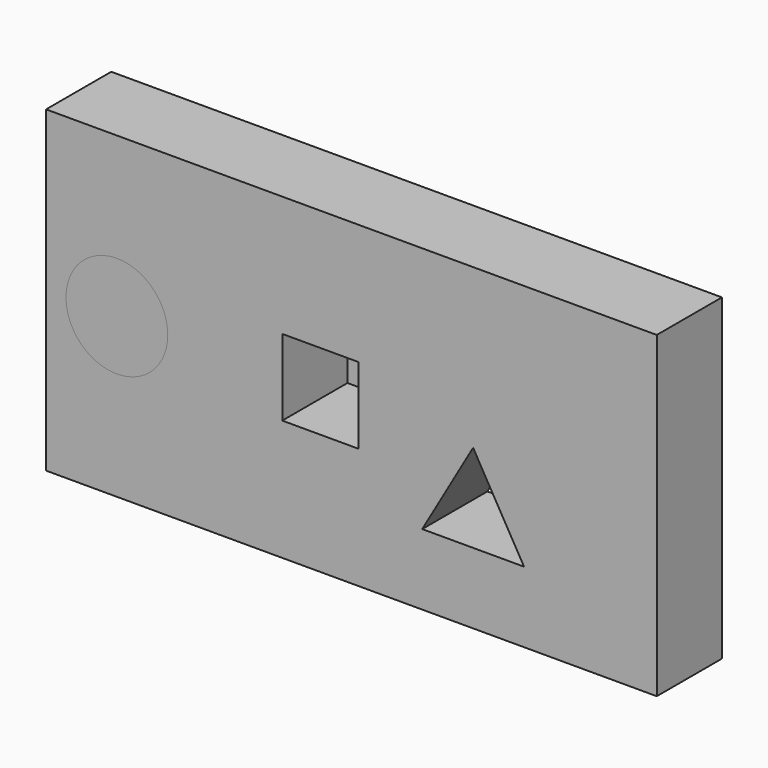
from build123d import *

# Parameters (mm, degrees)
F0_W     = 152.4
F0_H     = 79.375
F0_R     = 12.7
F0_W_2   = 19.05
F0_H_2   = 19.05
F1_DEPTH = 20.32
F2_DEPTH = 31.75
F3_DEPTH = 31.75
F4_DEPTH = 20.32


with BuildPart() as f1:
    # F0 (on Front) → F1 (new body)
    with BuildSketch(Plane.XZ):
        with Locations((-24.0162322402, 0)):
            Rectangle(F0_W, F0_H)
        Polygon((-6.35, -21.9970452561), (6.35, 0), (19.05, -21.9970452561), align=None, mode=Mode.SUBTRACT)
        with Locations((-82.55, 0)):
            Circle(F0_R, mode=Mode.SUBTRACT)
        with Locations((-31.75, 0)):
            Rectangle(F0_W_2, F0_H_2, mode=Mode.SUBTRACT)
    extrude(amount=F1_DEPTH)

    # F0 (on Front) → F2 (join)
    with BuildSketch(Plane.XZ):
        with Locations((-31.75, 0)):
            Rectangle(F0_W_2, F0_H_2)
    extrude(amount=-F2_DEPTH)

    # F0 (on Front) → F3 (join)
    with BuildSketch(Plane.XZ):
        with Locations((-82.55, 0)):
            Circle(F0_R)
    extrude(amount=-F3_DEPTH)


with BuildPart() as f4:
    # F4 (new): a face of the model
    f4_faces = [f1.part.faces().sort_by_distance(p)[0] for p in [
        (-82.55, 0, 0),
    ]]
    extrude(f4_faces, amount=F4_DEPTH)


solid = Compound([f1.part, f4.part])
